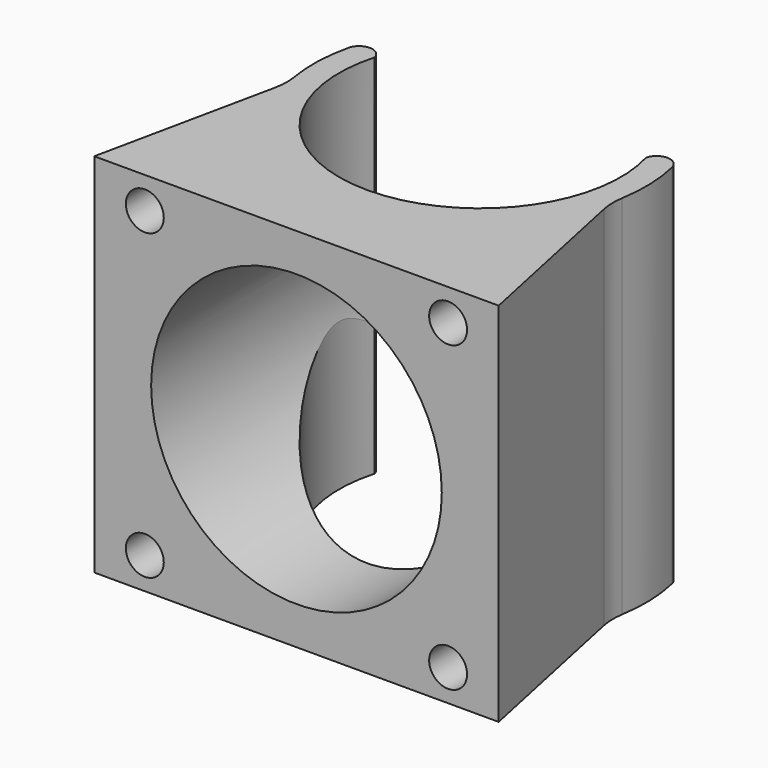
from build123d import *

# Parameters (mm, degrees)
F1_DEPTH = 29
F2_R     = 11.5
F3_DEPTH = 25
F2_R_2   = 1.5
F4_DEPTH = 8


# Not quite as in the source:
# - a feature names something its author has since deleted; it is built from what else it names


with BuildPart() as f1:
    # F0 (on Top) → F1 (new body)
    with BuildSketch(Plane.XY):
        with BuildLine():
            ThreePointArc((10.7388314076, 3), (0, -11.15), (-10.7388314076, 3))
            ThreePointArc((-10.7388314076, 3), (-11.7710268291, 3.8182927175), (-12.8032222507, 3))
            ThreePointArc((-12.8032222507, 3), (-13.142833705, 0.4340762628), (-12.9732702789, -2.148664299))
            ThreePointArc((-12.9732702789, -2.148664299), (-12.9072730339, -3.0752015435), (-13.0137997447, -3.9979577203))
            Line((-13.0137997447, -3.9979577203), (-16, -18.15))
            Line((-16, -18.15), (0, -18.15))
            Line((0, -18.15), (16, -18.15))
            Line((16, -18.15), (13.0137997447, -3.9979577203))
            ThreePointArc((13.0137997447, -3.9979577203), (12.9072730339, -3.0752015435), (12.9732702789, -2.148664299))
            ThreePointArc((12.9732702789, -2.148664299), (13.142833705, 0.4340762628), (12.8032222507, 3))
            ThreePointArc((12.8032222507, 3), (11.7710268291, 3.8182927175), (10.7388314076, 3))
        make_face()
    extrude(amount=F1_DEPTH)

    # F2 (on face) → F3 (cut)
    with BuildSketch(Plane.XZ.offset(18.15)):
        with Locations((0, 14.5)):
            Circle(F2_R)
    extrude(amount=-F3_DEPTH, mode=Mode.SUBTRACT)

    # F2 (on face) → F4 (cut)
    with BuildSketch(Plane.XZ.offset(18.15)):
        with Locations((-12, 26.5)):
            Circle(F2_R_2)
        with Locations((-12, 2.5)):
            Circle(F2_R_2)
        with Locations((12, 26.5)):
            Circle(F2_R_2)
        with Locations((12, 2.5)):
            Circle(F2_R_2)
    extrude(amount=-F4_DEPTH, mode=Mode.SUBTRACT)


solid = f1.part
